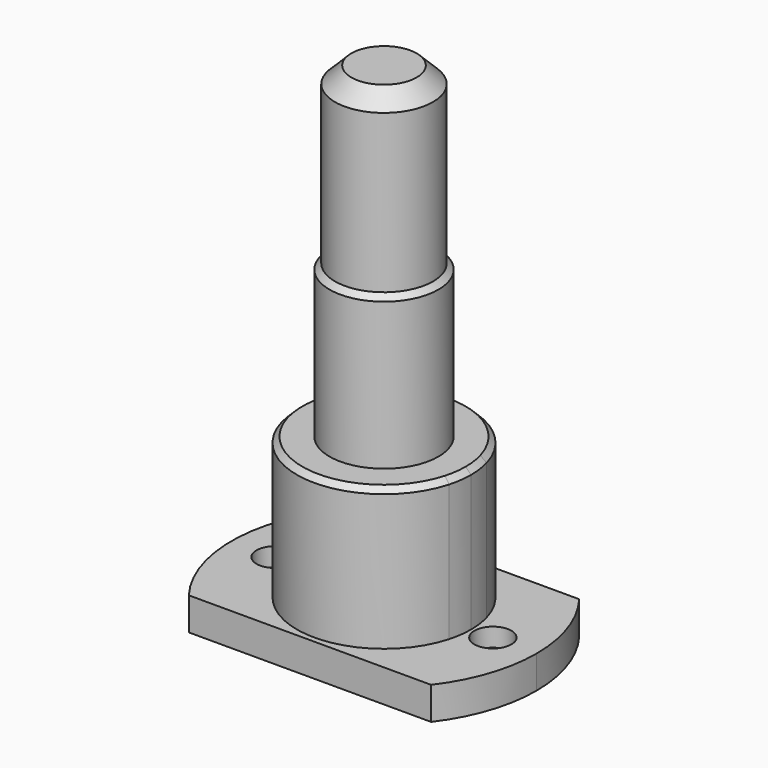
from build123d import *

# Parameters (mm, degrees)
F1_DEPTH        = 3
F2_DEPTH        = 16
F3_R            = 5
F4_DEPTH        = 14
F5_R            = 4.5
F6_DEPTH        = 16
F7_SIZE         = 1.5
F8_SIZE         = 0.49999
F9_D            = 3.4
F9_CSINK_D      = 6
F9_CSINK_ANGLE  = 90
F10_D           = 3.4
F10_CSINK_D     = 6
F10_CSINK_ANGLE = 90


# Not quite as in the source:
# - a fillet or chamfer is up to 0.001 mm smaller than in the source, because OpenCascade refuses the exact size


with BuildPart() as f1:
    # F0 (on Top) → F1 (new body)
    with BuildSketch(Plane.XY):
        with BuildLine():
            ThreePointArc((9.503875, 3.1106848096), (7.8523539336, 6.1919736516), (5.2411289459, 8.5164879717))
            Line((5.2411289459, 8.5164879717), (-5.2411289459, 8.5164879717))
            ThreePointArc((-5.2411289459, 8.5164879717), (-7.8523539336, 6.1919736516), (-9.503875, 3.1106848096))
            ThreePointArc((-9.503875, 3.1106848096), (-8.5246009554, 2.7831093509), (-7.703875, 2.15645774))
            ThreePointArc((-7.703875, 2.15645774), (0, 8), (7.703875, 2.15645774))
            ThreePointArc((7.703875, 2.15645774), (8.5246009554, 2.7831093509), (9.503875, 3.1106848096))
        make_face()
        with BuildLine():
            ThreePointArc((-7.703875, 2.15645774), (-8.5246009554, 2.7831093509), (-9.503875, 3.1106848096))
            ThreePointArc((-9.503875, 3.1106848096), (-9.705576078, 2.4086911373), (-9.8555, 1.6938476171))
            ThreePointArc((-9.8555, 1.6938476171), (-8.7478718117, 1.149858687), (-8.3, 0))
            ThreePointArc((-8.3, 0), (-8.7478718117, -1.149858687), (-9.8555, -1.6938476171))
            ThreePointArc((-9.8555, -1.6938476171), (-9.705576078, -2.4086911373), (-9.503875, -3.1106848096))
            ThreePointArc((-9.503875, -3.1106848096), (-8.5246009554, -2.7831093509), (-7.703875, -2.15645774))
            ThreePointArc((-7.703875, -2.15645774), (-8, 0), (-7.703875, 2.15645774))
        make_face()
        with BuildLine():
            ThreePointArc((-8.3, 0), (-8.7478718117, 1.149858687), (-9.8555, 1.6938476171))
            ThreePointArc((-9.8555, 1.6938476171), (-10, 0), (-9.8555, -1.6938476171))
            ThreePointArc((-9.8555, -1.6938476171), (-8.7478718117, -1.149858687), (-8.3, 0))
        make_face()
        with BuildLine():
            ThreePointArc((-9.8555, -1.6938476171), (-10, 0), (-9.8555, 1.6938476171))
            ThreePointArc((-9.8555, 1.6938476171), (-11.7, 0), (-9.8555, -1.6938476171))
        make_face()
        with BuildLine():
            ThreePointArc((-9.8555, 1.6938476171), (-9.705576078, 2.4086911373), (-9.503875, 3.1106848096))
            ThreePointArc((-9.503875, 3.1106848096), (-13.15, 0), (-9.503875, -3.1106848096))
            ThreePointArc((-9.503875, -3.1106848096), (-9.705576078, -2.4086911373), (-9.8555, -1.6938476171))
            ThreePointArc((-9.8555, -1.6938476171), (-11.7, 0), (-9.8555, 1.6938476171))
        make_face()
        with BuildLine():
            Line((-5.2411289459, 8.5164879717), (-11.1116800092, 8.5164879717))
            ThreePointArc((-11.1116800092, 8.5164879717), (-13.9999961512, 0.0103809935), (-11.1242977306, -8.5))
            Line((-11.1242977306, -8.5), (-5.2678268764, -8.5))
            ThreePointArc((-5.2678268764, -8.5), (-7.8620591219, -6.1796461357), (-9.503875, -3.1106848096))
            ThreePointArc((-9.503875, -3.1106848096), (-13.15, 0), (-9.503875, 3.1106848096))
            ThreePointArc((-9.503875, 3.1106848096), (-7.8523539336, 6.1919736516), (-5.2411289459, 8.5164879717))
        make_face()
        with BuildLine():
            ThreePointArc((11.1242977306, -8.5), (13.2616018683, -4.486637481), (14, 0))
            ThreePointArc((14, 0), (13.258271383, 4.4964697192), (11.1116800092, 8.5164879717))
            Line((11.1116800092, 8.5164879717), (5.2411289459, 8.5164879717))
            ThreePointArc((5.2411289459, 8.5164879717), (7.8523539336, 6.1919736516), (9.503875, 3.1106848096))
            ThreePointArc((9.503875, 3.1106848096), (12.0444689103, 2.3963820386), (13.15, 0))
            ThreePointArc((13.15, 0), (12.0444689103, -2.3963820386), (9.503875, -3.1106848096))
            ThreePointArc((9.503875, -3.1106848096), (7.8620591219, -6.1796461357), (5.2678268764, -8.5))
            Line((5.2678268764, -8.5), (11.1242977306, -8.5))
        make_face()
        with BuildLine():
            ThreePointArc((11.7, 0), (11.149858687, 1.2521281883), (9.8555, 1.6938476171))
            ThreePointArc((9.8555, 1.6938476171), (9.9638095124, 0.85), (10, 0))
            ThreePointArc((10, 0), (9.9638095124, -0.85), (9.8555, -1.6938476171))
            ThreePointArc((9.8555, -1.6938476171), (11.149858687, -1.2521281883), (11.7, 0))
        make_face()
        with BuildLine():
            ThreePointArc((13.15, 0), (12.0444689103, 2.3963820386), (9.503875, 3.1106848096))
            ThreePointArc((9.503875, 3.1106848096), (9.705576078, 2.4086911373), (9.8555, 1.6938476171))
            ThreePointArc((9.8555, 1.6938476171), (11.149858687, 1.2521281883), (11.7, 0))
            ThreePointArc((11.7, 0), (11.149858687, -1.2521281883), (9.8555, -1.6938476171))
            ThreePointArc((9.8555, -1.6938476171), (9.705576078, -2.4086911373), (9.503875, -3.1106848096))
            ThreePointArc((9.503875, -3.1106848096), (12.0444689103, -2.3963820386), (13.15, 0))
        make_face()
        with BuildLine():
            ThreePointArc((10, 0), (9.9638095124, 0.85), (9.8555, 1.6938476171))
            ThreePointArc((9.8555, 1.6938476171), (8.3, 0), (9.8555, -1.6938476171))
            ThreePointArc((9.8555, -1.6938476171), (9.9638095124, -0.85), (10, 0))
        make_face()
        with BuildLine():
            ThreePointArc((9.8555, 1.6938476171), (9.705576078, 2.4086911373), (9.503875, 3.1106848096))
            ThreePointArc((9.503875, 3.1106848096), (8.5246009554, 2.7831093509), (7.703875, 2.15645774))
            ThreePointArc((7.703875, 2.15645774), (7.9256230039, 1.088347371), (8, 0))
            ThreePointArc((8, 0), (7.9256230039, -1.088347371), (7.703875, -2.15645774))
            ThreePointArc((7.703875, -2.15645774), (8.5246009554, -2.7831093509), (9.503875, -3.1106848096))
            ThreePointArc((9.503875, -3.1106848096), (9.705576078, -2.4086911373), (9.8555, -1.6938476171))
            ThreePointArc((9.8555, -1.6938476171), (8.3, 0), (9.8555, 1.6938476171))
        make_face()
        with BuildLine():
            Line((-5.2678268764, -8.5), (5.2678268764, -8.5))
            ThreePointArc((5.2678268764, -8.5), (7.8620591219, -6.1796461357), (9.503875, -3.1106848096))
            ThreePointArc((9.503875, -3.1106848096), (8.5246009554, -2.7831093509), (7.703875, -2.15645774))
            ThreePointArc((7.703875, -2.15645774), (0, -8), (-7.703875, -2.15645774))
            ThreePointArc((-7.703875, -2.15645774), (-8.5246009554, -2.7831093509), (-9.503875, -3.1106848096))
            ThreePointArc((-9.503875, -3.1106848096), (-7.8620591219, -6.1796461357), (-5.2678268764, -8.5))
        make_face()
        with BuildLine():
            ThreePointArc((7.703875, -2.15645774), (6.85, 0), (7.703875, 2.15645774))
            ThreePointArc((7.703875, 2.15645774), (0, 8), (-7.703875, 2.15645774))
            ThreePointArc((-7.703875, 2.15645774), (-7.0712379962, 1.1596780264), (-6.85, 0))
            ThreePointArc((-6.85, 0), (-7.0712379962, -1.1596780264), (-7.703875, -2.15645774))
            ThreePointArc((-7.703875, -2.15645774), (0, -8), (7.703875, -2.15645774))
        make_face()
        with BuildLine():
            ThreePointArc((8, 0), (7.9256230039, 1.088347371), (7.703875, 2.15645774))
            ThreePointArc((7.703875, 2.15645774), (6.85, 0), (7.703875, -2.15645774))
            ThreePointArc((7.703875, -2.15645774), (7.9256230039, -1.088347371), (8, 0))
        make_face()
        with BuildLine():
            ThreePointArc((-6.85, 0), (-7.0712379962, 1.1596780264), (-7.703875, 2.15645774))
            ThreePointArc((-7.703875, 2.15645774), (-8, 0), (-7.703875, -2.15645774))
            ThreePointArc((-7.703875, -2.15645774), (-7.0712379962, -1.1596780264), (-6.85, 0))
        make_face()
    extrude(amount=F1_DEPTH)

    # F0 (on Top) → F2 (join)
    with BuildSketch(Plane.XY):
        with BuildLine():
            ThreePointArc((7.703875, -2.15645774), (6.85, 0), (7.703875, 2.15645774))
            ThreePointArc((7.703875, 2.15645774), (0, 8), (-7.703875, 2.15645774))
            ThreePointArc((-7.703875, 2.15645774), (-7.0712379962, 1.1596780264), (-6.85, 0))
            ThreePointArc((-6.85, 0), (-7.0712379962, -1.1596780264), (-7.703875, -2.15645774))
            ThreePointArc((-7.703875, -2.15645774), (0, -8), (7.703875, -2.15645774))
        make_face()
        with BuildLine():
            ThreePointArc((-6.85, 0), (-7.0712379962, 1.1596780264), (-7.703875, 2.15645774))
            ThreePointArc((-7.703875, 2.15645774), (-8, 0), (-7.703875, -2.15645774))
            ThreePointArc((-7.703875, -2.15645774), (-7.0712379962, -1.1596780264), (-6.85, 0))
        make_face()
        with BuildLine():
            ThreePointArc((8, 0), (7.9256230039, 1.088347371), (7.703875, 2.15645774))
            ThreePointArc((7.703875, 2.15645774), (6.85, 0), (7.703875, -2.15645774))
            ThreePointArc((7.703875, -2.15645774), (7.9256230039, -1.088347371), (8, 0))
        make_face()
    extrude(amount=F2_DEPTH)

    # F3 (on face) → F4 (join)
    with BuildSketch(Plane.XY.offset(16)):
        Circle(F3_R)
    extrude(amount=F4_DEPTH)

    # F5 (on face) → F6 (join)
    with BuildSketch(Plane.XY.offset(30)):
        Circle(F5_R)
    extrude(amount=F6_DEPTH)

    # F7
    f7_edges = [f1.edges().sort_by_distance(p)[0] for p in [
        (-4.5, 0, 46),
    ]]
    chamfer(f7_edges, length=F7_SIZE)

    # F8 (size 0.5 in the source; OpenCascade refuses exactly that, so slightly less here)
    f8_edges = [f1.edges().sort_by_distance(p)[0] for p in [
        (-7.703875, 2.156458, 16),
        (-5, 0, 30),
    ]]
    chamfer(f8_edges, length=F8_SIZE)

    # F9 (through all)
    with Locations(Plane(origin=(0, 0, 0), x_dir=(1, 0, 0), z_dir=(0, 0, -1))):
        with Locations((10, 0)):
            CounterSinkHole(F9_D / 2, F9_CSINK_D / 2, counter_sink_angle=F9_CSINK_ANGLE)

    # F10 (through all)
    with Locations(Plane(origin=(0, 0, 0), x_dir=(1, 0, 0), z_dir=(0, 0, -1))):
        with Locations((-10, 0)):
            CounterSinkHole(F10_D / 2, F10_CSINK_D / 2, counter_sink_angle=F10_CSINK_ANGLE)


solid = f1.part
